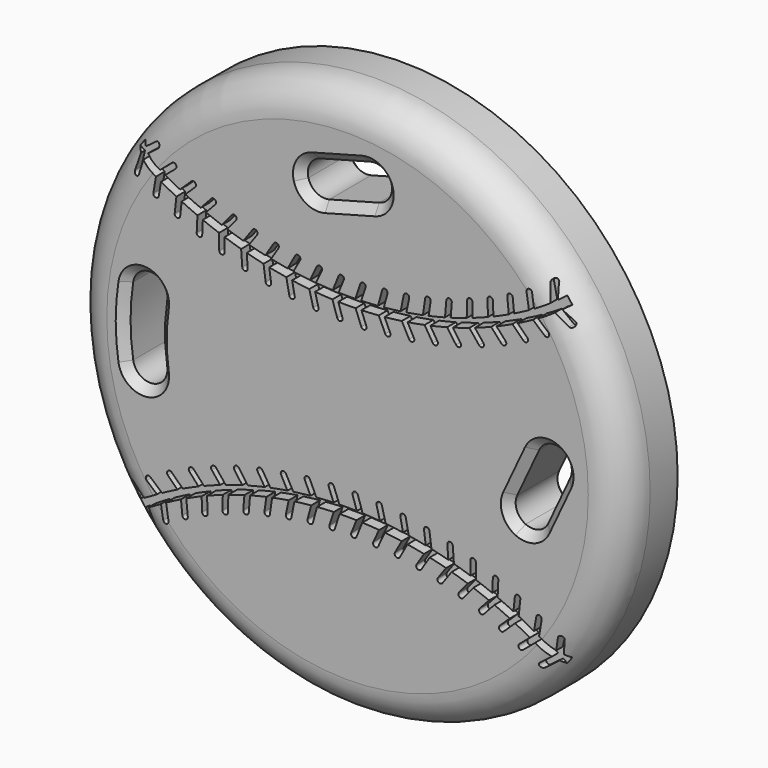
from build123d import *

# Parameters (mm, degrees)
F0_R      = 12.7
F1_DEPTH  = 3.175
F2_SIZE   = 0.381
F5_DEPTH  = 0.508
F7_DEPTH  = 0.508
F9_DEPTH  = 0.508
F14_DEPTH = 25.4
F15_SIZE  = 0.381
F17_DEPTH = 25.4
F18_SIZE  = 0.381


# Not quite as in the source:
# - ends of sketch curves that miss each other by under 0.0002 mm in the source are joined


with BuildPart() as f1:
    # F0 (on Front) → F1 (new body)
    with BuildSketch(Plane.XZ):
        Circle(F0_R)
        with BuildLine():
            ThreePointArc((-10.1959033593, -1.5875), (-10.31875, 0), (-10.1959033593, 1.5875))
            ThreePointArc((-10.1959033593, 1.5875), (-9.2894877163, 2.2496848738), (-8.6273028425, 1.3432692308))
            ThreePointArc((-8.6273028425, 1.3432692308), (-8.73125, 0), (-8.6273028425, -1.3432692308))
            ThreePointArc((-8.6273028425, -1.3432692308), (-9.2894877163, -2.2496848738), (-10.1959033593, -1.5875))
        make_face(mode=Mode.SUBTRACT)
    extrude(amount=F1_DEPTH)

    # F2
    f2_edges = [f1.edges().sort_by_distance(p)[0] for p in [
        (-9.289488, -3.175, -2.249685),
        (-8.73125, -3.175, 0),
        (-8.73125, 0, 0),
    ]]
    chamfer(f2_edges, length=F2_SIZE)

    # F4 (on face) → F5 (cut)
    with BuildSketch(Plane.XZ.offset(3.175)):
        with BuildLine():
            ThreePointArc((10.0903170963, 7.7120361057), (0, 4.4873333333), (-10.0903170963, 7.7120361057))
            ThreePointArc((-10.0903170963, 7.7120361057), (-10.204882315, 7.5597868314), (-10.3171505, 7.4058359123))
            ThreePointArc((-10.3171505, 7.4058359123), (0, 4.1063333333), (10.3171505, 7.4058359123))
            ThreePointArc((10.3171505, 7.4058359123), (10.204882315, 7.5597868314), (10.0903170963, 7.7120361057))
        make_face()
        with BuildLine():
            ThreePointArc((-10.3171505, -7.4058359123), (-10.204882315, -7.5597868314), (-10.0903170963, -7.7120361057))
            ThreePointArc((-10.0903170963, -7.7120361057), (0, -4.4873333333), (10.0903170963, -7.7120361057))
            ThreePointArc((10.0903170963, -7.7120361057), (10.204882315, -7.5597868314), (10.3171505, -7.4058359123))
            ThreePointArc((10.3171505, -7.4058359123), (0, -4.1063333333), (-10.3171505, -7.4058359123))
        make_face()
    extrude(amount=-F5_DEPTH, mode=Mode.SUBTRACT)

    # F6 (on face) → F7 (cut)
    with BuildSketch(Plane.XZ.offset(3.175)):
        with BuildLine():
            Line((8.9655202832, -7.7774051542), (9.7084275034, -7.2188150469))
            ThreePointArc((9.7084275034, -7.2188150469), (9.5954418436, -7.1446517893), (9.481889674, -7.0713588641))
            Line((9.481889674, -7.0713588641), (8.8128738495, -7.5743902131))
            ThreePointArc((8.8128738495, -7.5743902131), (8.7876895958, -7.7522209005), (8.9655202832, -7.7774051542))
        make_face()
        with BuildLine():
            Line((-9.1205047211, -7.8770944945), (-9.3207214809, -6.9694341534))
            ThreePointArc((-9.3207214809, -6.9694341534), (-9.4350615627, -7.0414917261), (-9.5488446034, -7.1144257218))
            Line((-9.5488446034, -7.1144257218), (-9.3685418994, -7.931807913))
            ThreePointArc((-9.3685418994, -7.931807913), (-9.217166601, -8.0284697929), (-9.1205047211, -7.8770944945))
        make_face()
        with BuildLine():
            ThreePointArc((-9.5488446034, -7.1144257218), (-9.4350615627, -7.0414917261), (-9.3207214809, -6.9694341534))
            Line((-9.3207214809, -6.9694341534), (-10.0499520862, -6.4086497383))
            ThreePointArc((-10.0499520862, -6.4086497383), (-10.2280453511, -6.4319046086), (-10.2047904808, -6.6099978735))
            Line((-10.2047904808, -6.6099978735), (-9.5488446034, -7.1144257218))
        make_face()
        with BuildLine():
            Line((-8.2616111371, -7.3540137205), (-8.4068864974, -6.4359564699))
            ThreePointArc((-8.4068864974, -6.4359564699), (-8.5253526153, -6.5010081955), (-8.6433154009, -6.5669682539))
            Line((-8.6433154009, -6.5669682539), (-8.5124894884, -7.3937132522))
            ThreePointArc((-8.5124894884, -7.3937132522), (-8.3672005469, -7.4993026621), (-8.2616111371, -7.3540137205))
        make_face()
        with BuildLine():
            ThreePointArc((-8.6433154009, -6.5669682539), (-8.5253526153, -6.5010081955), (-8.4068864974, -6.4359564699))
            Line((-8.4068864974, -6.4359564699), (-9.1010766453, -5.8323369918))
            ThreePointArc((-9.1010766453, -5.8323369918), (-9.280245996, -5.8448407425), (-9.2677422452, -6.0240100932))
            Line((-9.2677422452, -6.0240100932), (-8.6433154009, -6.5669682539))
        make_face()
        with BuildLine():
            Line((-7.3728180575, -6.8835261579), (-7.4626262541, -5.9583945275))
            ThreePointArc((-7.4626262541, -5.9583945275), (-7.5847896689, -6.0162049781), (-7.7065052817, -6.0749523839))
            Line((-7.7065052817, -6.0749523839), (-7.6256296312, -6.9080681266))
            ThreePointArc((-7.6256296312, -6.9080681266), (-7.48695286, -7.0222029291), (-7.3728180575, -6.8835261579))
        make_face()
        with BuildLine():
            ThreePointArc((-7.7065052817, -6.0749523839), (-7.5847896689, -6.0162049781), (-7.4626262541, -5.9583945275))
            Line((-7.4626262541, -5.9583945275), (-8.1192636096, -5.3141245382))
            ThreePointArc((-8.1192636096, -5.3141245382), (-8.2988606164, -5.3158319172), (-8.2971532374, -5.495428924))
            Line((-8.2971532374, -5.495428924), (-7.7065052817, -6.0749523839))
        make_face()
        with BuildLine():
            Line((-6.4573421027, -6.4673345424), (-6.4913581118, -5.5384766648))
            ThreePointArc((-6.4913581118, -5.5384766648), (-6.6167767033, -5.5888366191), (-6.7418046438, -5.6401587604))
            Line((-6.7418046438, -5.6401587604), (-6.7111719514, -6.4766301285))
            ThreePointArc((-6.7111719514, -6.4766301285), (-6.5796092339, -6.5988972598), (-6.4573421027, -6.4673345424))
        make_face()
        with BuildLine():
            ThreePointArc((-6.7418046438, -5.6401587604), (-6.6167767033, -5.5888366191), (-6.4913581118, -5.5384766648))
            Line((-6.4913581118, -5.5384766648), (-7.1080662467, -4.8558878338))
            ThreePointArc((-7.1080662467, -4.8558878338), (-7.2874409323, -4.8467926619), (-7.2965361041, -5.0261673476))
            Line((-7.2965361041, -5.0261673476), (-6.7418046438, -5.6401587604))
        make_face()
        with BuildLine():
            Line((-5.5184964603, -6.1069451079), (-5.4965971749, -5.1777226012))
            ThreePointArc((-5.4965971749, -5.1777226012), (-5.6248170423, -5.2204498023), (-5.7527048234, -5.2641609397))
            Line((-5.7527048234, -5.2641609397), (-5.7724259515, -6.10096067))
            ThreePointArc((-5.7724259515, -6.10096067), (-5.6484534248, -6.2309176346), (-5.5184964603, -6.1069451079))
        make_face()
        with BuildLine():
            ThreePointArc((-5.7527048234, -5.2641609397), (-5.6248170423, -5.2204498023), (-5.4965971749, -5.1777226012))
            Line((-5.4965971749, -5.1777226012), (-6.0711441684, -4.4592852774))
            ThreePointArc((-6.0711441684, -4.4592852774), (-6.2496473602, -4.439420471), (-6.2695121666, -4.6179236627))
            Line((-6.2695121666, -4.6179236627), (-5.7527048234, -5.2641609397))
        make_face()
        with BuildLine():
            Line((-4.559678895, -5.8036621355), (-4.4819435707, -4.8774379374))
            ThreePointArc((-4.4819435707, -4.8774379374), (-4.612500675, -4.9123777518), (-4.7427854596, -4.9483196908))
            Line((-4.7427854596, -4.9483196908), (-4.8127890357, -5.7824193317))
            ThreePointArc((-4.8127890357, -5.7824193317), (-4.6968553672, -5.9195958039), (-4.559678895, -5.8036621355))
        make_face()
        with BuildLine():
            ThreePointArc((-4.7427854596, -4.9483196908), (-4.612500675, -4.9123777518), (-4.4819435707, -4.8774379374))
            Line((-4.4819435707, -4.8774379374), (-5.0122500868, -4.1257522086))
            ThreePointArc((-5.0122500868, -4.1257522086), (-5.1892357659, -4.09518966), (-5.2197983146, -4.2721753391))
            Line((-5.2197983146, -4.2721753391), (-4.7427854596, -4.9483196908))
        make_face()
        with BuildLine():
            Line((-3.5843594519, -5.5585832327), (-3.4510694196, -4.63870943))
            ThreePointArc((-3.4510694196, -4.63870943), (-3.5834912631, -4.6657354074), (-3.7157015392, -4.6937780711))
            Line((-3.7157015392, -4.6937780711), (-3.8357342141, -5.5221589427))
            ThreePointArc((-3.8357342141, -5.5221589427), (-3.728258978, -5.6660584689), (-3.5843594519, -5.5585832327))
        make_face()
        with BuildLine():
            ThreePointArc((-3.7157015392, -4.6937780711), (-3.5834912631, -4.6657354074), (-3.4510694196, -4.63870943))
            Line((-3.4510694196, -4.63870943), (-3.9352162324, -3.8564957127))
            ThreePointArc((-3.9352162324, -3.8564957127), (-4.1100438722, -3.8153460305), (-4.1511935545, -3.9901736703))
            Line((-4.1511935545, -3.9901736703), (-3.7157015392, -4.6937780711))
        make_face()
        with BuildLine():
            Line((-2.5960678974, -5.3725953618), (-2.4077055454, -4.4624010583))
            ThreePointArc((-2.4077055454, -4.4624010583), (-2.541512882, -4.4814153893), (-2.6751701689, -4.5014572888))
            Line((-2.6751701689, -4.5014572888), (-2.8447975339, -5.3211214082))
            ThreePointArc((-2.8447975339, -5.3211214082), (-2.7461696925, -5.4712232033), (-2.5960678974, -5.3725953618))
        make_face()
        with BuildLine():
            ThreePointArc((-2.6751701689, -4.5014572888), (-2.541512882, -4.4814153893), (-2.4077055454, -4.4624010583))
            Line((-2.4077055454, -4.4624010583), (-2.8439404852, -3.6524902526))
            ThreePointArc((-2.8439404852, -3.6524902526), (-3.0159773692, -3.6009023611), (-3.0675652608, -3.772939245))
            Line((-3.0675652608, -3.772939245), (-2.6751701689, -4.5014572888))
        make_face()
        with BuildLine():
            Line((-1.5983809455, -5.246371629), (-1.3556279737, -4.3491508979))
            ThreePointArc((-1.3556279737, -4.3491508979), (-1.4903365427, -4.360084768), (-1.6249571231, -4.3720533698))
            Line((-1.6249571231, -4.3720533698), (-1.8435652819, -5.1800343006))
            ThreePointArc((-1.8435652819, -5.1800343006), (-1.7541417779, -5.335795133), (-1.5983809455, -5.246371629))
        make_face()
        with BuildLine():
            ThreePointArc((-1.6249571231, -4.3720533698), (-1.4903365427, -4.360084768), (-1.3556279737, -4.3491508979))
            Line((-1.3556279737, -4.3491508979), (-1.742372268, -3.514474142))
            ThreePointArc((-1.742372268, -3.514474142), (-1.9109957795, -3.4526347423), (-1.9728351792, -3.6212582538))
            Line((-1.9728351792, -3.6212582538), (-1.6249571231, -4.3720533698))
        make_face()
        with BuildLine():
            Line((-0.5949093127, -5.1803688492), (-0.2986442654, -4.2993688109))
            ThreePointArc((-0.2986442654, -4.2993688109), (-0.4337665448, -4.3021826495), (-0.5688632149, -4.3060346383))
            Line((-0.5688632149, -4.3060346383), (-0.8356610054, -5.0994082266))
            ThreePointArc((-0.8356610054, -5.0994082266), (-0.7557654704, -5.2602643843), (-0.5949093127, -5.1803688492))
        make_face()
        with BuildLine():
            ThreePointArc((-0.5688632149, -4.3060346383), (-0.4337665448, -4.3021826495), (-0.2986442654, -4.2993688109))
            Line((-0.2986442654, -4.2993688109), (-0.6344982526, -3.4429468734))
            ThreePointArc((-0.6344982526, -3.4429468734), (-0.7990981284, -3.3710797676), (-0.8709652341, -3.5356796434))
            Line((-0.8709652341, -3.5356796434), (-0.5688632149, -4.3060346383))
        make_face()
        with BuildLine():
            Line((0.4107153491, -5.1748258922), (0.7594202627, -4.3132349632))
            ThreePointArc((0.7594202627, -4.3132349632), (0.6243732923, -4.3079185867), (0.4892894591, -4.3036400218))
            Line((0.4892894591, -4.3036400218), (0.1752676015, -5.0795349789))
            ThreePointArc((0.1752676015, -5.0795349789), (0.2453460187, -5.2449043094), (0.4107153491, -5.1748258922))
        make_face()
        with BuildLine():
            ThreePointArc((0.4892894591, -4.3036400218), (0.6243732923, -4.3079185867), (0.7594202627, -4.3132349632))
            Line((0.7594202627, -4.3132349632), (0.4756720676, -3.43816731))
            ThreePointArc((0.4756720676, -3.43816731), (0.3156915289, -3.3565325916), (0.2340568106, -3.5165131303))
            Line((0.2340568106, -3.5165131303), (0.4892894591, -4.3036400218))
        make_face()
        with BuildLine():
            Line((1.414853596, -5.2297628184), (1.8147363823, -4.3906991719))
            ThreePointArc((1.8147363823, -4.3906991719), (1.6802534676, -4.3772718207), (1.5456713517, -4.3648781866))
            Line((1.5456713517, -4.3648781866), (1.1855618997, -5.1204864807))
            ThreePointArc((1.1855618997, -5.1204864807), (1.245569579, -5.2897704977), (1.414853596, -5.2297628184))
        make_face()
        with BuildLine():
            ThreePointArc((1.5456713517, -4.3648781866), (1.6802534676, -4.3772718207), (1.8147363823, -4.3906991719))
            Line((1.8147363823, -4.3906991719), (1.5841208889, -3.5001527497))
            ThreePointArc((1.5841208889, -3.5001527497), (1.4293386709, -3.4090458619), (1.3382317831, -3.5638280798))
            Line((1.3382317831, -3.5638280798), (1.5456713517, -4.3648781866))
        make_face()
        with BuildLine():
            Line((2.4138713637, -5.3449808064), (2.8634848117, -4.5314810872))
            ThreePointArc((2.8634848117, -4.5314810872), (2.7300526583, -4.5099913561), (2.5964593241, -4.4895275065))
            Line((2.5964593241, -4.4895275065), (2.1915655453, -5.2221145249))
            ThreePointArc((2.1915655453, -5.2221145249), (2.2412853137, -5.3947005748), (2.4138713637, -5.3449808064))
        make_face()
        with BuildLine():
            ThreePointArc((2.5964593241, -4.4895275065), (2.7300526583, -4.5099913561), (2.8634848117, -4.5314810872))
            Line((2.8634848117, -4.5314810872), (2.6868366377, -3.6286788616))
            ThreePointArc((2.6868366377, -3.6286788616), (2.5378129109, -3.5284295282), (2.4375635775, -3.677453255))
            Line((2.4375635775, -3.677453255), (2.5964593241, -4.4895275065))
        make_face()
        with BuildLine():
            Line((3.4041531191, -5.520062872), (3.9018700383, -4.7350712071))
            ThreePointArc((3.9018700383, -4.7350712071), (3.7699715489, -4.7055968693), (3.6378504824, -4.6771368646))
            Line((3.6378504824, -4.6771368646), (3.189637723, -5.3840513105))
            ThreePointArc((3.189637723, -5.3840513105), (3.2288896403, -5.5593147893), (3.4041531191, -5.520062872))
        make_face()
        with BuildLine():
            ThreePointArc((3.6378504824, -4.6771368646), (3.7699715489, -4.7055968693), (3.9018700383, -4.7350712071))
            Line((3.9018700383, -4.7350712071), (3.779828489, -3.8232804985))
            ThreePointArc((3.779828489, -3.8232804985), (3.6371025833, -3.7142515307), (3.5280736154, -3.8569774364))
            Line((3.5280736154, -3.8569774364), (3.6378504824, -4.6771368646))
        make_face()
        with BuildLine():
            Line((4.3821149457, -5.7543753779), (4.926134055, -5.0007327209))
            ThreePointArc((4.926134055, -5.0007327209), (4.7962465817, -4.9633804468), (4.6660759406, -4.9270272862))
            Line((4.6660759406, -4.9270272862), (4.1761663219, -5.6057107743))
            ThreePointArc((4.1761663219, -5.6057107743), (4.204808332, -5.783017388), (4.3821149457, -5.7543753779))
        make_face()
        with BuildLine():
            ThreePointArc((4.6660759406, -4.9270272862), (4.7962465817, -4.9633804468), (4.926134055, -5.0007327209))
            Line((4.926134055, -5.0007327209), (4.8591408094, -4.0832533801))
            ThreePointArc((4.8591408094, -4.0832533801), (4.7232292623, -3.9658393631), (4.6058152454, -4.1017509102))
            Line((4.6058152454, -4.1017509102), (4.6660759406, -4.9270272862))
        make_face()
        with BuildLine():
            Line((5.3442175139, -6.0470703267), (5.9325699604, -5.3275041765))
            ThreePointArc((5.9325699604, -5.3275041765), (5.8051635774, -5.2824091471), (5.6774144607, -5.2382943959))
            Line((5.6774144607, -5.2382943959), (5.1475810086, -5.8862907112))
            ThreePointArc((5.1475810086, -5.8862907112), (5.1655094535, -6.0649987716), (5.3442175139, -6.0470703267))
        make_face()
        with BuildLine():
            ThreePointArc((5.6774144607, -5.2382943959), (5.8051635774, -5.2824091471), (5.9325699604, -5.3275041765))
            Line((5.9325699604, -5.3275041765), (5.9208674729, -4.4076566415))
            ThreePointArc((5.9208674729, -4.4076566415), (5.7922621603, -4.2822825071), (5.6668880259, -4.4108878197))
            Line((5.6668880259, -4.4108878197), (5.6774144607, -5.2382943959))
        make_face()
        with BuildLine():
            Line((6.2869788901, -6.3970884296), (6.9175353746, -5.7142029593))
            ThreePointArc((6.9175353746, -5.7142029593), (6.7930711768, -5.6615283774), (6.6682059198, -5.6098116908))
            Line((6.6682059198, -5.6098116908), (6.100366148, -6.2247756777))
            ThreePointArc((6.100366148, -6.2247756777), (6.1075161431, -6.4042384247), (6.2869788901, -6.3970884296))
        make_face()
        with BuildLine():
            ThreePointArc((6.6682059198, -5.6098116908), (6.7930711768, -5.6615283774), (6.9175353746, -5.7142029593))
            Line((6.9175353746, -5.7142029593), (6.9611659976, -4.7953162391))
            ThreePointArc((6.9611659976, -4.7953162391), (6.8403323534, -4.6624357272), (6.7074518416, -4.7832693714))
            Line((6.7074518416, -4.7832693714), (6.6682059198, -5.6098116908))
        make_face()
        with BuildLine():
            Line((7.2069871381, -6.8031629404), (7.8774656214, -6.1594295724))
            ThreePointArc((7.8774656214, -6.1594295724), (7.7563940557, -6.099366072), (7.6348645567, -6.0402346172))
            Line((7.6348645567, -6.0402346172), (7.0310735271, -6.619940667))
            ThreePointArc((7.0310735271, -6.619940667), (7.0274191959, -6.7995086092), (7.2069871381, -6.8031629404))
        make_face()
        with BuildLine():
            ThreePointArc((7.6348645567, -6.0402346172), (7.7563940557, -6.099366072), (7.8774656214, -6.1594295724))
            Line((7.8774656214, -6.1594295724), (7.9762714519, -5.2448291986))
            ThreePointArc((7.9762714519, -5.2448291986), (7.8636467837, -5.1049232155), (7.7237408006, -5.2175478837))
            Line((7.7237408006, -5.2175478837), (7.6348645567, -6.0402346172))
        make_face()
        with BuildLine():
            Line((8.1009126675, -7.2638242398), (8.8088866291, -6.6615727016))
            ThreePointArc((8.8088866291, -6.6615727016), (8.6916458641, -6.5943376578), (8.5738919489, -6.5280054368))
            Line((8.5738919489, -6.5280054368), (7.9363348343, -7.0703555425))
            ThreePointArc((7.9363348343, -7.0703555425), (7.9218894022, -7.2493788077), (8.1009126675, -7.2638242398))
        make_face()
        with BuildLine():
            ThreePointArc((8.5738919489, -6.5280054368), (8.6916458641, -6.5943376578), (8.8088866291, -6.6615727016))
            Line((8.8088866291, -6.6615727016), (8.9625100801, -5.7545686932))
            ThreePointArc((8.9625100801, -5.7545686932), (8.8585019863, -5.6081435709), (8.7120768641, -5.7121516647))
            Line((8.7120768641, -5.7121516647), (8.5738919489, -6.5280054368))
        make_face()
        with BuildLine():
            ThreePointArc((9.481889674, -7.0713588641), (9.5954418436, -7.1446517893), (9.7084275034, -7.2188150469))
            Line((9.7084275034, -7.2188150469), (9.916312598, -6.322689931))
            ThreePointArc((9.916312598, -6.322689931), (9.8212974932, -6.1702755949), (9.6688831571, -6.2652906998))
            Line((9.6688831571, -6.2652906998), (9.481889674, -7.0713588641))
        make_face()
    extrude(amount=-F7_DEPTH, mode=Mode.SUBTRACT)

    # F8 (on face) → F9 (cut)
    with BuildSketch(Plane.XZ.offset(3.175)):
        with BuildLine():
            Line((-8.9656531004, 7.7774905851), (-9.7085603205, 7.2189004778))
            ThreePointArc((-9.7085603205, 7.2189004778), (-9.5955741895, 7.1447379357), (-9.4820226835, 7.0714439946))
            Line((-9.4820226835, 7.0714439946), (-8.8130066667, 7.574475644))
            ThreePointArc((-8.8130066667, 7.574475644), (-8.787822413, 7.7523063314), (-8.9656531004, 7.7774905851))
        make_face()
        with BuildLine():
            ThreePointArc((-9.4820226835, 7.0714439946), (-9.5955741895, 7.1447379357), (-9.7085591779, 7.218902204))
            Line((-9.7085591779, 7.218902204), (-9.9164454152, 6.3227753619))
            ThreePointArc((-9.9164454152, 6.3227753619), (-9.8214303103, 6.1703610258), (-9.6690159742, 6.2653761307))
            Line((-9.6690159742, 6.2653761307), (-9.4820226835, 7.0714439946))
        make_face()
        with BuildLine():
            Line((9.1205047211, 7.8770944945), (9.3207214809, 6.9694341534))
            ThreePointArc((9.3207214809, 6.9694341534), (9.4350615627, 7.0414917261), (9.5488446034, 7.1144257218))
            Line((9.5488446034, 7.1144257218), (9.3685418994, 7.931807913))
            ThreePointArc((9.3685418994, 7.931807913), (9.217166601, 8.0284697929), (9.1205047211, 7.8770944945))
        make_face()
        with BuildLine():
            ThreePointArc((9.5488446034, 7.1144257218), (9.4350615627, 7.0414917261), (9.3207214809, 6.9694341534))
            Line((9.3207214809, 6.9694341534), (10.0499520862, 6.4086497383))
            ThreePointArc((10.0499520862, 6.4086497383), (10.2280453511, 6.4319046086), (10.2047904808, 6.6099978735))
            Line((10.2047904808, 6.6099978735), (9.5488446034, 7.1144257218))
        make_face()
        with BuildLine():
            Line((8.2616023603, 7.3540139847), (8.4068777206, 6.435956734))
            ThreePointArc((8.4068777206, 6.435956734), (8.5253460125, 6.5010045368), (8.6433088565, 6.5669645615))
            Line((8.6433088565, 6.5669645615), (8.5124807117, 7.3937135163))
            ThreePointArc((8.5124807117, 7.3937135163), (8.3671917702, 7.4993029262), (8.2616023603, 7.3540139847))
        make_face()
        with BuildLine():
            ThreePointArc((8.6433088565, 6.5669645615), (8.5253460125, 6.5010045368), (8.4068798364, 6.4359528455))
            Line((8.4068798364, 6.4359528455), (9.1010678685, 5.8323372559))
            ThreePointArc((9.1010678685, 5.8323372559), (9.2802372192, 5.8448410067), (9.2677334684, 6.0240103573))
            Line((9.2677334684, 6.0240103573), (8.6433088565, 6.5669645615))
        make_face()
        with BuildLine():
            Line((7.3728005358, 6.8835272134), (7.4626087323, 5.9583955831))
            ThreePointArc((7.4626087323, 5.9583955831), (7.5847758163, 6.0161983575), (7.7064915391, 6.0749456857))
            Line((7.7064915391, 6.0749456857), (7.6256121094, 6.9080691821))
            ThreePointArc((7.6256121094, 6.9080691821), (7.4869353383, 7.0222039846), (7.3728005358, 6.8835272134))
        make_face()
        with BuildLine():
            ThreePointArc((7.7064915391, 6.0749456857), (7.5847758163, 6.0161983575), (7.4626122919, 5.9583879858))
            Line((7.4626122919, 5.9583879858), (8.1192460879, 5.3141255937))
            ThreePointArc((8.1192460879, 5.3141255937), (8.2988430947, 5.3158329727), (8.2971357156, 5.4954299795))
            Line((8.2971357156, 5.4954299795), (7.7064915391, 6.0749456857))
        make_face()
        with BuildLine():
            Line((6.4573158993, 6.4673369137), (6.4913319084, 5.5384790361))
            ThreePointArc((6.4913319084, 5.5384790361), (6.6167550351, 5.5888278218), (6.7417831294, 5.6401498324))
            Line((6.7417831294, 5.6401498324), (6.711145748, 6.4766324999))
            ThreePointArc((6.711145748, 6.4766324999), (6.5795830306, 6.5988996311), (6.4573158993, 6.4673369137))
        make_face()
        with BuildLine():
            ThreePointArc((6.7417831294, 5.6401498324), (6.6167550351, 5.5888278218), (6.4913362906, 5.538468))
            Line((6.4913362906, 5.538468), (7.1080400433, 4.8558902051))
            ThreePointArc((7.1080400433, 4.8558902051), (7.287414729, 4.8467950333), (7.2965099008, 5.0261697189))
            Line((7.2965099008, 5.0261697189), (6.7417831294, 5.6401498324))
        make_face()
        with BuildLine():
            Line((5.5184616702, 6.1069493147), (5.4965623848, 5.177726808))
            ThreePointArc((5.4965623848, 5.177726808), (5.6247870854, 5.2204396916), (5.7526750548, 5.2641506371))
            Line((5.7526750548, 5.2641506371), (5.7723911614, 6.1009648768))
            ThreePointArc((5.7723911614, 6.1009648768), (5.6484186347, 6.2309218414), (5.5184616702, 6.1069493147))
        make_face()
        with BuildLine():
            ThreePointArc((5.7526750548, 5.2641506371), (5.6247870854, 5.2204396916), (5.496567031, 5.1777126847))
            Line((5.496567031, 5.1777126847), (6.0711093783, 4.4592894842))
            ThreePointArc((6.0711093783, 4.4592894842), (6.2496125701, 4.4394246778), (6.2694773765, 4.6179278695))
            Line((6.2694773765, 4.6179278695), (5.7526750548, 5.2641506371))
        make_face()
        with BuildLine():
            Line((4.5596356441, 5.8036686908), (4.4819003198, 4.8774444927))
            ThreePointArc((4.4819003198, 4.8774444927), (4.6124620582, 4.912367258), (4.7427470553, 4.9483089373))
            Line((4.7427470553, 4.9483089373), (4.8127457847, 5.782425887))
            ThreePointArc((4.8127457847, 5.782425887), (4.6968121163, 5.9196023592), (4.5596356441, 5.8036686908))
        make_face()
        with BuildLine():
            ThreePointArc((4.7427470553, 4.9483089373), (4.6124620582, 4.912367258), (4.4819047432, 4.8774277061))
            Line((4.4819047432, 4.8774277061), (5.0122068359, 4.1257587639))
            ThreePointArc((5.0122068359, 4.1257587639), (5.189192515, 4.0951962153), (5.2197550636, 4.2721818944))
            Line((5.2197550636, 4.2721818944), (4.7427470553, 4.9483089373))
        make_face()
        with BuildLine():
            Line((3.5843078966, 5.5585926411), (3.4510178643, 4.6387188383))
            ThreePointArc((3.4510178643, 4.6387188383), (3.5834437256, 4.6657255151), (3.7156542272, 4.6937678458))
            Line((3.7156542272, 4.6937678458), (3.8356826588, 5.522168351))
            ThreePointArc((3.8356826588, 5.522168351), (3.7282074227, 5.6660678772), (3.5843078966, 5.5585926411))
        make_face()
        with BuildLine():
            ThreePointArc((3.7156542272, 4.6937678458), (3.5834437256, 4.6657255151), (3.4510216589, 4.6386998736))
            Line((3.4510216589, 4.6386998736), (3.9351646771, 3.856505121))
            ThreePointArc((3.9351646771, 3.856505121), (4.109992317, 3.8153554388), (4.1511419992, 3.9901830786))
            Line((4.1511419992, 3.9901830786), (3.7156542272, 4.6937678458))
        make_face()
        with BuildLine():
            Line((2.5960082244, 5.3726081173), (2.4076458724, 4.4624138138))
            ThreePointArc((2.4076458724, 4.4624138138), (2.5414562801, 4.4814071242), (2.6751137936, 4.5014486138))
            Line((2.6751137936, 4.5014486138), (2.8447378609, 5.3211341637))
            ThreePointArc((2.8447378609, 5.3211341637), (2.7461100195, 5.4712359588), (2.5960082244, 5.3726081173))
        make_face()
        with BuildLine():
            ThreePointArc((2.6751137936, 4.5014486138), (2.5414562801, 4.4814071242), (2.40764872, 4.462393206))
            Line((2.40764872, 4.462393206), (2.8438808122, 3.6525030081))
            ThreePointArc((2.8438808122, 3.6525030081), (3.0159176962, 3.6009151166), (3.0675055878, 3.7729520006))
            Line((3.0675055878, 3.7729520006), (2.6751137936, 4.5014486138))
        make_face()
        with BuildLine():
            Line((1.5983133707, 5.2463882138), (1.3555603989, 4.3491674827))
            ThreePointArc((1.3555603989, 4.3491674827), (1.4902708551, 4.3600791823), (1.6248916506, 4.3720472954))
            Line((1.6248916506, 4.3720472954), (1.8434977072, 5.1800508854))
            ThreePointArc((1.8434977072, 5.1800508854), (1.7540742031, 5.3358117178), (1.5983133707, 5.2463882138))
        make_face()
        with BuildLine():
            ThreePointArc((1.6248916506, 4.3720472954), (1.4902708551, 4.3600791823), (1.3555620746, 4.3491458039))
            Line((1.3555620746, 4.3491458039), (1.7423046932, 3.5144907268))
            ThreePointArc((1.7423046932, 3.5144907268), (1.9109282047, 3.4526513271), (1.9727676045, 3.6212748386))
            Line((1.9727676045, 3.6212748386), (1.6248916506, 4.3720472954))
        make_face()
        with BuildLine():
            Line((0.5948340807, 5.1803897315), (0.2985690334, 4.2993896932))
            ThreePointArc((0.2985690334, 4.2993896932), (0.4336918755, 4.3021808077), (0.5687887366, 4.3060322285))
            Line((0.5687887366, 4.3060322285), (0.8355857735, 5.0994291088))
            ThreePointArc((0.8355857735, 5.0994291088), (0.7556902384, 5.2602852666), (0.5948340807, 5.1803897315))
        make_face()
        with BuildLine():
            ThreePointArc((0.5687887366, 4.3060322285), (0.4336918755, 4.3021808077), (0.2985694095, 4.2993675399))
            Line((0.2985694095, 4.2993675399), (0.6344230206, 3.4429677556))
            ThreePointArc((0.6344230206, 3.4429677556), (0.7990228964, 3.3711006499), (0.8708900022, 3.5357005257))
            Line((0.8708900022, 3.5357005257), (0.5687887366, 4.3060322285))
        make_face()
        with BuildLine():
            Line((-0.4107979661, 5.1748515246), (-0.7595028797, 4.3132605956))
            ThreePointArc((-0.7595028797, 4.3132605956), (-0.624456712, 4.3079215499), (-0.489372725, 4.3036423391))
            Line((-0.489372725, 4.3036423391), (-0.1753502185, 5.0795606114))
            ThreePointArc((-0.1753502185, 5.0795606114), (-0.2454286356, 5.2449299418), (-0.4107979661, 5.1748515246))
        make_face()
        with BuildLine():
            ThreePointArc((-0.489372725, 4.3036423391), (-0.624456712, 4.3079215499), (-0.7595038314, 4.3132385748))
            Line((-0.7595038314, 4.3132385748), (-0.4757546845, 3.4381929424))
            ThreePointArc((-0.4757546845, 3.4381929424), (-0.3157741459, 3.3565582241), (-0.2341394275, 3.5165387627))
            Line((-0.2341394275, 3.5165387627), (-0.489372725, 4.3036423391))
        make_face()
        with BuildLine():
            Line((-1.4149432989, 5.2297936365), (-1.8148260852, 4.3907299899))
            ThreePointArc((-1.8148260852, 4.3907299899), (-1.6803452798, 4.3772806318), (-1.5457630596, 4.364886277))
            Line((-1.5457630596, 4.364886277), (-1.1856516026, 5.1205172988))
            ThreePointArc((-1.1856516026, 5.1205172988), (-1.2456592819, 5.2898013158), (-1.4149432989, 5.2297936365))
        make_face()
        with BuildLine():
            ThreePointArc((-1.5457630596, 4.364886277), (-1.6803452798, 4.3772806318), (-1.814828293, 4.3907087056))
            Line((-1.814828293, 4.3907087056), (-1.5842105917, 3.5001835677))
            ThreePointArc((-1.5842105917, 3.5001835677), (-1.4294283738, 3.4090766799), (-1.338321486, 3.5638588979))
            Line((-1.338321486, 3.5638588979), (-1.5457630596, 4.364886277))
        make_face()
        with BuildLine():
            Line((-2.4139678278, 5.3450172268), (-2.8635812758, 4.5315175076))
            ThreePointArc((-2.8635812758, 4.5315175076), (-2.7301523801, 4.5100070242), (-2.5965590036, 4.489542384))
            Line((-2.5965590036, 4.489542384), (-2.1916620095, 5.2221509453))
            ThreePointArc((-2.1916620095, 5.2221509453), (-2.2413817779, 5.3947369952), (-2.4139678278, 5.3450172268))
        make_face()
        with BuildLine():
            ThreePointArc((-2.5965590036, 4.489542384), (-2.7301523801, 4.5100070242), (-2.8635845694, 4.5314975473))
            Line((-2.8635845694, 4.5314975473), (-2.6869331018, 3.628715282))
            ThreePointArc((-2.6869331018, 3.628715282), (-2.537909375, 3.5284659486), (-2.4376600416, 3.6774896754))
            Line((-2.4376600416, 3.6774896754), (-2.5965590036, 4.489542384))
        make_face()
        with BuildLine():
            Line((-3.4042559954, 5.5201052911), (-3.9019729147, 4.7351136262))
            ThreePointArc((-3.9019729147, 4.7351136262), (-3.7700785767, 4.705620355), (-3.6379575417, 4.6771594964))
            Line((-3.6379575417, 4.6771594964), (-3.1897405993, 5.3840937297))
            ThreePointArc((-3.1897405993, 5.3840937297), (-3.2289925167, 5.5593572085), (-3.4042559954, 5.5201052911))
        make_face()
        with BuildLine():
            ThreePointArc((-3.6379575417, 4.6771594964), (-3.7700785767, 4.705620355), (-3.9019770277, 4.7350955474))
            Line((-3.9019770277, 4.7350955474), (-3.7799313653, 3.8233229177))
            ThreePointArc((-3.7799313653, 3.8233229177), (-3.6372054596, 3.7142939498), (-3.5281764917, 3.8570198555))
            Line((-3.5281764917, 3.8570198555), (-3.6379575417, 4.6771594964))
        make_face()
        with BuildLine():
            Line((-4.3822238619, 5.7544241706), (-4.9262429712, 5.0007815136))
            ThreePointArc((-4.9262429712, 5.0007815136), (-4.7963601968, 4.9634126479), (-4.666189672, 4.9270585782))
            Line((-4.666189672, 4.9270585782), (-4.1762752381, 5.605759567))
            ThreePointArc((-4.1762752381, 5.605759567), (-4.2049172482, 5.7830661806), (-4.3822238619, 5.7544241706))
        make_face()
        with BuildLine():
            ThreePointArc((-4.666189672, 4.9270585782), (-4.7963601968, 4.9634126479), (-4.9262475465, 5.0007658312))
            Line((-4.9262475465, 5.0007658312), (-4.8592497256, 4.0833021727))
            ThreePointArc((-4.8592497256, 4.0833021727), (-4.7233381785, 3.9658881558), (-4.6059241616, 4.1017997028))
            Line((-4.6059241616, 4.1017997028), (-4.666189672, 4.9270585782))
        make_face()
        with BuildLine():
            Line((-5.3443320758, 6.0471258445), (-5.9326845223, 5.3275596943))
            ThreePointArc((-5.9326845223, 5.3275596943), (-5.8052829534, 5.2824508849), (-5.6775340477, 5.238335179))
            Line((-5.6775340477, 5.238335179), (-5.1476955705, 5.8863462289))
            ThreePointArc((-5.1476955705, 5.8863462289), (-5.1656240154, 6.0650542894), (-5.3443320758, 6.0471258445))
        make_face()
        with BuildLine():
            ThreePointArc((-5.6775340477, 5.238335179), (-5.8052829534, 5.2824508849), (-5.9326891177, 5.3275468682))
            Line((-5.9326891177, 5.3275468682), (-5.9209820348, 4.4077121593))
            ThreePointArc((-5.9209820348, 4.4077121593), (-5.7923767222, 4.2823380249), (-5.6670025878, 4.4109433375))
            Line((-5.6670025878, 4.4109433375), (-5.6775340477, 5.238335179))
        make_face()
        with BuildLine():
            Line((-6.2870986831, 6.3971509998), (-6.9176551676, 5.7142655295))
            ThreePointArc((-6.9176551676, 5.7142655295), (-6.7931953885, 5.6615803839), (-6.668330446, 5.6098627081))
            Line((-6.668330446, 5.6098627081), (-6.100485941, 6.2248382479))
            ThreePointArc((-6.100485941, 6.2248382479), (-6.1076359361, 6.4043009949), (-6.2870986831, 6.3971509998))
        make_face()
        with BuildLine():
            ThreePointArc((-6.668330446, 5.6098627081), (-6.7931953885, 5.6615803839), (-6.9176592639, 5.7142559533))
            Line((-6.9176592639, 5.7142559533), (-6.9612857906, 4.7953788093))
            ThreePointArc((-6.9612857906, 4.7953788093), (-6.8404521464, 4.6624982974), (-6.7075716346, 4.7833319416))
            Line((-6.7075716346, 4.7833319416), (-6.668330446, 5.6098627081))
        make_face()
        with BuildLine():
            Line((-7.2071117287, 6.8032328649), (-7.877590212, 6.1594994968))
            ThreePointArc((-7.877590212, 6.1594994968), (-7.7565220898, 6.0994289785), (-7.6349930162, 6.040296512))
            Line((-7.6349930162, 6.040296512), (-7.0311981176, 6.6200105915))
            ThreePointArc((-7.0311981176, 6.6200105915), (-7.0275437865, 6.7995785337), (-7.2071117287, 6.8032328649))
        make_face()
        with BuildLine():
            ThreePointArc((-7.6349930162, 6.040296512), (-7.7565220898, 6.0994289785), (-7.8775932221, 6.1594934876))
            Line((-7.8775932221, 6.1594934876), (-7.9763960425, 5.244899123))
            ThreePointArc((-7.9763960425, 5.244899123), (-7.8637713742, 5.10499314), (-7.7238653911, 5.2176178082))
            Line((-7.7238653911, 5.2176178082), (-7.6349930162, 6.040296512))
        make_face()
        with BuildLine():
            Line((-8.1010416046, 7.2639017937), (-8.8090155663, 6.6616502555))
            ThreePointArc((-8.8090155663, 6.6616502555), (-8.6917766307, 6.5944119842), (-8.5740232578, 6.5280787423))
            Line((-8.5740232578, 6.5280787423), (-7.9364637715, 7.0704330964))
            ThreePointArc((-7.9364637715, 7.0704330964), (-7.9220183394, 7.2494563616), (-8.1010416046, 7.2639017937))
        make_face()
        with BuildLine():
            ThreePointArc((-8.5740232578, 6.5280787423), (-8.6917766307, 6.5944119842), (-8.8090168454, 6.6616480448))
            Line((-8.8090168454, 6.6616480448), (-8.9626390173, 5.7546462471))
            ThreePointArc((-8.9626390173, 5.7546462471), (-8.8586309235, 5.6082211248), (-8.7122058012, 5.7122292186))
            Line((-8.7122058012, 5.7122292186), (-8.5740232578, 6.5280787423))
        make_face()
    extrude(amount=-F9_DEPTH, mode=Mode.SUBTRACT)

    # F10 (on Top) → F12 (revolve, cut)
    with BuildSketch(Plane.XY):
        with BuildLine():
            ThreePointArc((-11.1125, -3.175), (-12.2350320151, -2.7100320151), (-12.7, -1.5875))
            Line((-12.7, -1.5875), (-12.7, -3.175))
            Line((-12.7, -3.175), (-11.1125, -3.175))
        make_face()
    revolve(axis=Axis((0, -1.5875, 0), (0, -1, 0)), mode=Mode.SUBTRACT)

    # F13 (on face) → F14 (cut)
    with BuildSketch(Plane.XZ.offset(3.175)):
        with BuildLine():
            ThreePointArc((9.5924371272, 1.2294557845), (8.9855053932, 1.2559549963), (8.537602076, 0.8455272238))
            Line((8.537602076, 0.8455272238), (7.5312423402, -1.312618194))
            ThreePointArc((7.5312423402, -1.312618194), (7.5047431284, -1.9195499281), (7.9151709009, -2.3674532453))
            ThreePointArc((7.9151709009, -2.3674532453), (8.5221026349, -2.393952457), (8.9700059521, -1.9835246846))
            Line((8.9700059521, -1.9835246846), (9.9763656879, 0.1746207333))
            ThreePointArc((9.9763656879, 0.1746207333), (10.0028648997, 0.7815524673), (9.5924371272, 1.2294557845))
        make_face()
    extrude(amount=-F14_DEPTH, mode=Mode.SUBTRACT)

    # F15
    f15_edges = [f1.edges().sort_by_distance(p)[0] for p in [
        (8.034422, -3.175, -0.233545),
        (8.034422, 0, -0.233545),
    ]]
    chamfer(f15_edges, length=F15_SIZE)

    # F16 (on face) → F17 (cut)
    with BuildSketch(Plane.XZ.offset(3.175)):
        with BuildLine():
            Line((0.7509392644, 10.0331956077), (-1.5491716095, 9.4168827566))
            ThreePointArc((-1.5491716095, 9.4168827566), (-2.0311416567, 9.047054132), (-2.1104376171, 8.4447415149))
            ThreePointArc((-2.1104376171, 8.4447415149), (-1.7406089924, 7.9627714677), (-1.1382963754, 7.8834755073))
            Line((-1.1382963754, 7.8834755073), (1.1618144985, 8.4997883585))
            ThreePointArc((1.1618144985, 8.4997883585), (1.6437845457, 8.8696169831), (1.723080506, 9.4719296002))
            ThreePointArc((1.723080506, 9.4719296002), (1.3532518814, 9.9538996474), (0.7509392644, 10.0331956077))
        make_face()
    extrude(amount=-F17_DEPTH, mode=Mode.SUBTRACT)

    # F18
    f18_edges = [f1.edges().sort_by_distance(p)[0] for p in [
        (0.011759, -3.175, 8.191632),
        (1.161814, -1.5875, 8.499788),
        (0.011759, 0, 8.191632),
        (-1.138296, -1.5875, 7.883476),
    ]]
    chamfer(f18_edges, length=F18_SIZE)


solid = f1.part
